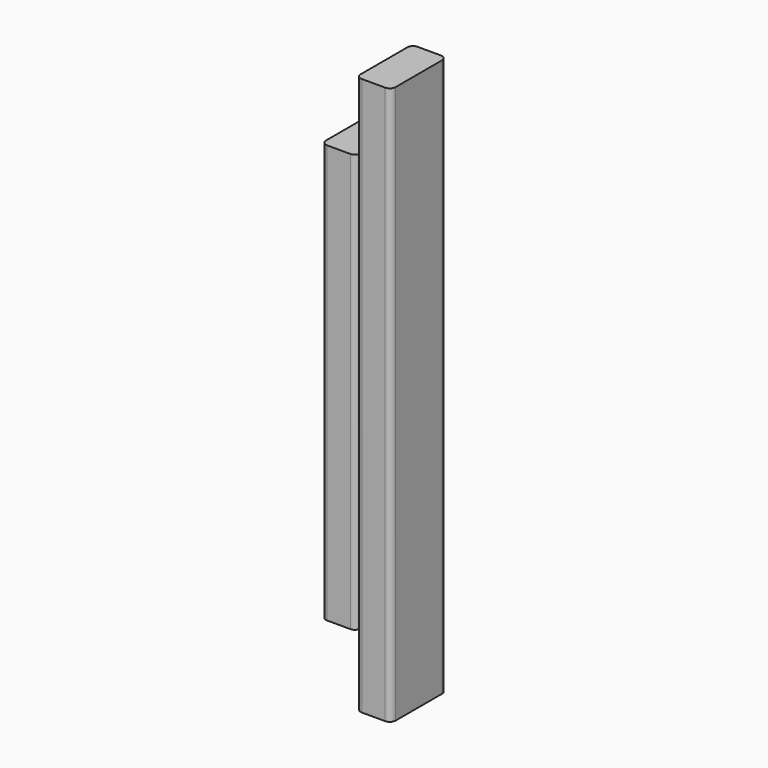
from build123d import *

# Parameters (mm, degrees)
F1_DEPTH = 304.8
F2_DEPTH = 266.7
F3_DEPTH = 38.1


# Not quite as in the source:
# - a feature names something its author has since deleted; it is built from what else it names


with BuildPart() as f1:
    # F0 (on Top) → F1 (new body)
    with BuildSketch(Plane.XY):
        with BuildLine():
            Line((19.05, 34.9504), (19.05, 3.1496))
            ThreePointArc((19.05, 3.1496), (19.972496482, 0.922496482), (22.1996, 0))
            Line((22.1996, 0), (34.9504, 0))
            ThreePointArc((34.9504, 0), (37.177503518, 0.922496482), (38.1, 3.1496))
            Line((38.1, 3.1496), (38.1, 34.9504))
            ThreePointArc((38.1, 34.9504), (37.177503518, 37.177503518), (34.9504, 38.1))
            Line((34.9504, 38.1), (22.1996, 38.1))
            ThreePointArc((22.1996, 38.1), (19.972496482, 37.177503518), (19.05, 34.9504))
        make_face()
    extrude(amount=F1_DEPTH)

    # F0 (on Top) → F2 (join)
    with BuildSketch(Plane.XY):
        with BuildLine():
            ThreePointArc((0, 3.1496), (0.922496482, 0.922496482), (3.1496, 0))
            Line((3.1496, 0), (15.9004, 0))
            ThreePointArc((15.9004, 0), (18.127503518, 0.922496482), (19.05, 3.1496))
            Line((19.05, 3.1496), (19.05, 34.9504))
            ThreePointArc((19.05, 34.9504), (18.127503518, 37.177503518), (15.9004, 38.1))
            Line((15.9004, 38.1), (3.1496, 38.1))
            ThreePointArc((3.1496, 38.1), (0.922496482, 37.177503518), (0, 34.9504))
            Line((0, 34.9504), (0, 3.1496))
        make_face()
        with BuildLine():
            Line((19.05, 34.9504), (19.05, 3.1496))
            ThreePointArc((19.05, 3.1496), (19.972496482, 0.922496482), (22.1996, 0))
            Line((22.1996, 0), (34.9504, 0))
            ThreePointArc((34.9504, 0), (37.177503518, 0.922496482), (38.1, 3.1496))
            Line((38.1, 3.1496), (38.1, 34.9504))
            ThreePointArc((38.1, 34.9504), (37.177503518, 37.177503518), (34.9504, 38.1))
            Line((34.9504, 38.1), (22.1996, 38.1))
            ThreePointArc((22.1996, 38.1), (19.972496482, 37.177503518), (19.05, 34.9504))
        make_face()
    extrude(amount=F2_DEPTH)

    # F0 (on Top) → F3 (cut)
    with BuildSketch(Plane.XY):
        with BuildLine():
            ThreePointArc((0, 3.1496), (0.922496482, 0.922496482), (3.1496, 0))
            Line((3.1496, 0), (15.9004, 0))
            ThreePointArc((15.9004, 0), (18.127503518, 0.922496482), (19.05, 3.1496))
            Line((19.05, 3.1496), (19.05, 34.9504))
            ThreePointArc((19.05, 34.9504), (18.127503518, 37.177503518), (15.9004, 38.1))
            Line((15.9004, 38.1), (3.1496, 38.1))
            ThreePointArc((3.1496, 38.1), (0.922496482, 37.177503518), (0, 34.9504))
            Line((0, 34.9504), (0, 3.1496))
        make_face()
    extrude(amount=F3_DEPTH, mode=Mode.SUBTRACT)


solid = f1.part
